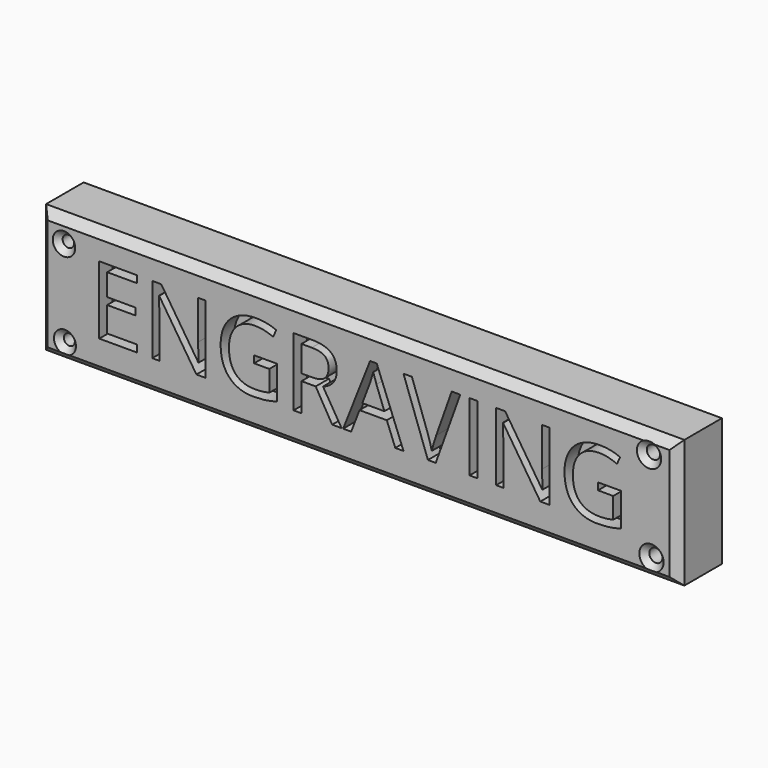
from build123d import *

# Parameters (mm, degrees)
F0_W         = 231.2171161175
F0_H         = 46.4802645147
F1_DEPTH     = 20
F3_TEXT_SIZE = 34.5394752609
F4_DEPTH     = 6
F5_R         = 2.6479744649
F6_DEPTH     = 25
F7_R         = 2.0723678172
F8_DEPTH     = 25
F9_R         = 1.99055402
F10_DEPTH    = 25
F11_R        = 2.3923481952
F12_DEPTH    = 25
F13_R        = 2.3923481952
F14_DEPTH    = 25
F15_SIZE     = 2
F16_SIZE     = 2
F17_SIZE     = 2
F18_SIZE     = 2
F19_T1_DEPTH = 246.6472140453
F19_T3_DEPTH = 61.9103624425


# Not quite as in the source:
# - a fillet or chamfer that OpenCascade refuses, or shapes differently, is made with other operations: its cross-section is extruded or revolved along the edge and cut away or added
# - Text() gives the source's letters only with a copy of the font that has no kerning and outlines rounded to 1/6400 em; it was checked with that copy


with BuildPart() as f1:
    # F0 (on Front) → F1 (new body)
    with BuildSketch(Plane.XZ):
        Rectangle(F0_W, F0_H)
    extrude(amount=F1_DEPTH)

    # F3 (on offset) → F4 (cut)
    with BuildSketch(Plane.XZ.offset(20)):
        with Locations((-97.3392571162, -11.3980267197)):
            Text('ENGRAVING', F3_TEXT_SIZE, font='Open Sans', text_align=(TextAlign.LEFT, TextAlign.BOTTOM))
    extrude(amount=-F4_DEPTH, mode=Mode.SUBTRACT)

    # F5 (on offset) → F6 (cut)
    with BuildSketch(Plane.XZ.offset(20)):
        with Locations((-105.8388203382, 15.5427642167)):
            Circle(F5_R)
    extrude(amount=F6_DEPTH, mode=Mode.SUBTRACT)

    # F7 (on Front) → F8 (cut)
    with BuildSketch(Plane.XZ):
        with Locations((-106.7269742489, 14.6546065807)):
            Circle(F7_R)
    extrude(amount=F8_DEPTH, mode=Mode.SUBTRACT)

    # F9 (on Front) → F10 (cut)
    with BuildSketch(Plane.XZ):
        with Locations((-106.379263103, -16.5927931666)):
            Circle(F9_R)
    extrude(amount=F10_DEPTH, mode=Mode.SUBTRACT)

    # F11 (on Front) → F12 (cut)
    with BuildSketch(Plane.XZ):
        with Locations((105.1923260093, 16.3447186351)):
            Circle(F11_R)
    extrude(amount=F12_DEPTH, mode=Mode.SUBTRACT)

    # F13 (on Front) → F14 (cut)
    with BuildSketch(Plane.XZ):
        with Locations((106.0825288296, -16.2960588932)):
            Circle(F13_R)
    extrude(amount=F14_DEPTH, mode=Mode.SUBTRACT)

    # F15
    f15_edges = [f1.edges().sort_by_distance(p)[0] for p in [
        (-108.799342, -20, 14.654607),
    ]]
    chamfer(f15_edges, length=F15_SIZE)

    # F16
    f16_edges = [f1.edges().sort_by_distance(p)[0] for p in [
        (-108.369817, -20, -16.592793),
    ]]
    chamfer(f16_edges, length=F16_SIZE)

    # F17
    f17_edges = [f1.edges().sort_by_distance(p)[0] for p in [
        (102.799978, -20, 16.344719),
    ]]
    chamfer(f17_edges, length=F17_SIZE)

    # F18
    f18_edges = [f1.edges().sort_by_distance(p)[0] for p in [
        (103.690181, -20, -16.296059),
    ]]
    chamfer(f18_edges, length=F18_SIZE)

    # F19: chamfer of 3 on 4 edges, made by hand

    # F19_s2 → F19_t1 (cut)
    with BuildSketch(Plane.YZ.offset(-123.3236070226)):
        Polygon((-20, 20.2401322573), (-17, 23.2401322573), (-20, 23.2401322573), align=None)
        Polygon((-20, -20.2401322573), (-17, -23.2401322573), (-20, -23.2401322573), align=None)
    extrude(amount=F19_T1_DEPTH, mode=Mode.SUBTRACT)

    # F19_s4 → F19_t3 (cut)
    with BuildSketch(Plane.XY.offset(-30.9551812212)):
        Polygon((-112.6085580587, -20), (-115.6085580587, -17), (-115.6085580587, -20), align=None)
        Polygon((112.6085580587, -20), (115.6085580587, -17), (115.6085580587, -20), align=None)
    extrude(amount=F19_T3_DEPTH, mode=Mode.SUBTRACT)


solid = f1.part
